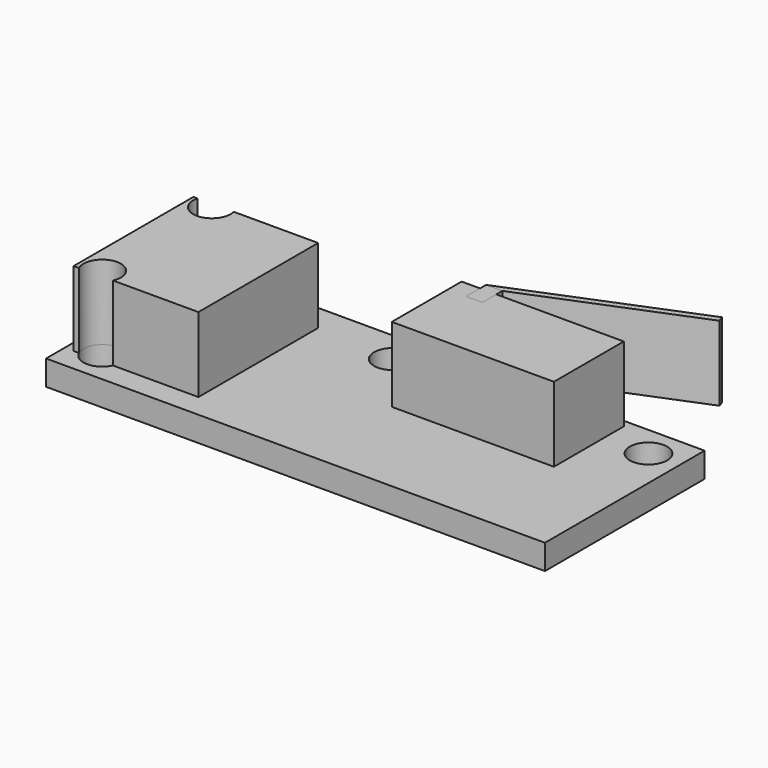
from build123d import *
from build123d import SkipClean  # not in build123d's __all__

# Parameters (mm, degrees)
F0_W     = 40
F0_H     = 16
F0_R     = 1.5
F1_DEPTH = 2
F3_DEPTH = 6
F4_DEPTH = 2


with BuildPart() as f1:
    # F0 (on Top) → F1 (new body)
    with BuildSketch(Plane.XY):
        with Locations((7.0192306489, 1.2307697609)):
            Rectangle(F0_W, F0_H)
        with Locations((-10.4807693511, -4.2692302391)):
            Circle(F0_R, mode=Mode.SUBTRACT)
        with Locations((-10.4807693511, 6.7307697609)):
            Circle(F0_R, mode=Mode.SUBTRACT)
        with Locations((4.0192306489, 6.7307697609)):
            Circle(F0_R, mode=Mode.SUBTRACT)
        with Locations((24.5192306489, 6.7307697609)):
            Circle(F0_R, mode=Mode.SUBTRACT)
    extrude(amount=F1_DEPTH)

    # F2 (on face) → F3 (join)
    with BuildSketch(Plane.XY.offset(2)):
        with BuildLine():
            Line((-11.9339417158, 7.102643501), (-12.2648915183, 7.102643501))
            Line((-12.2648915183, 7.102643501), (-12.2648915183, -4.897356499))
            Line((-12.2648915183, -4.897356499), (-11.8429211054, -4.897356499))
            ThreePointArc((-11.8429211054, -4.897356499), (-10.8023065718, -2.8040975435), (-8.9807693511, -4.2692302391))
            ThreePointArc((-8.9807693511, -4.2692302391), (-9.0156366555, -4.5907674598), (-9.1186175969, -4.897356499))
            Line((-9.1186175969, -4.897356499), (-2.2648915183, -4.897356499))
            Line((-2.2648915183, -4.897356499), (-2.2648915183, 7.102643501))
            Line((-2.2648915183, 7.102643501), (-9.0275969865, 7.102643501))
            ThreePointArc((-9.0275969865, 7.102643501), (-8.9925223039, 6.9181750076), (-8.9807693511, 6.7307697609))
            ThreePointArc((-8.9807693511, 6.7307697609), (-10.6681745979, 5.2425227137), (-11.9339417158, 7.102643501))
        make_face()
        Polygon((9.3223992735, 8.6297835391), (8.0192306489, 8.6297835391), (8.0192306489, 1.6297835391), (21.0192306489, 1.6297835391), (21.0192306489, 8.6297835391), align=None)
        Polygon((23.7675364597, 15.032194342), (9.4975042399, 9.2307697609), (10.8031475786, 9.2307697609), (23.9558426598, 14.569008877), align=None)
    with SkipClean():  # cleaning this boolean's faces spoils the solid; the shape is the same uncleaned
        extrude(amount=F3_DEPTH)


with BuildPart() as f4:
    # F4 (new): a face of the model
    f4_faces = [f1.part.faces().sort_by_distance(p)[0] for p in [
        (10.1503259093, 9.2307697609, 5),
    ]]
    extrude(f4_faces, amount=F4_DEPTH)


solid = Compound([f1.part, f4.part])
